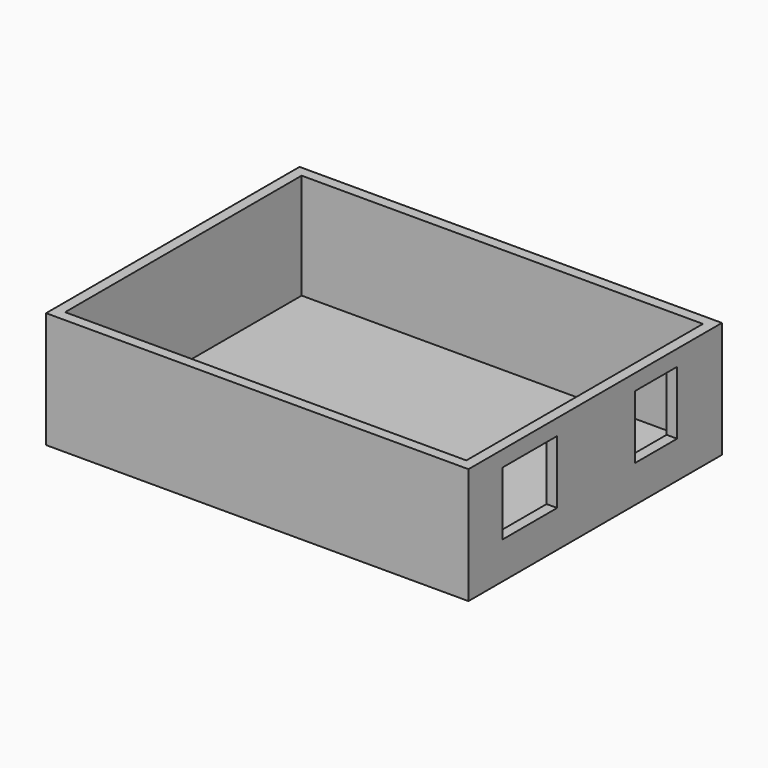
from build123d import *

# Parameters (mm, degrees)
F0_W     = 80
F0_H     = 60
F1_DEPTH = 2
F2_W     = 80
F2_H     = 60
F2_W_2   = 76
F2_H_2   = 56
F3_DEPTH = 20
F4_W     = 13
F4_H     = 12
F4_W_2   = 10
F5_DEPTH = 2


# Not quite as in the source:
# - the program builds the solid bodies; features that only make, move or delete a surface that nothing else refers to are left out


with BuildPart() as f1:
    # F0 (on Top) → F1 (new body)
    with BuildSketch(Plane.XY):
        Rectangle(F0_W, F0_H)
    extrude(amount=F1_DEPTH)

    # F2 (on face) → F3 (join)
    with BuildSketch(Plane.XY.offset(2)):
        Rectangle(F2_W, F2_H)
        Rectangle(F2_W_2, F2_H_2, mode=Mode.SUBTRACT)
    extrude(amount=F3_DEPTH)

    # F4 (on face) → F5 (cut)
    with BuildSketch(Plane.YZ.offset(40)):
        with Locations((-15.5, 13)):
            Rectangle(F4_W, F4_H)
        with Locations((14.4, 13)):
            Rectangle(F4_W_2, F4_H)
    extrude(amount=-F5_DEPTH, mode=Mode.SUBTRACT)


solid = f1.part
